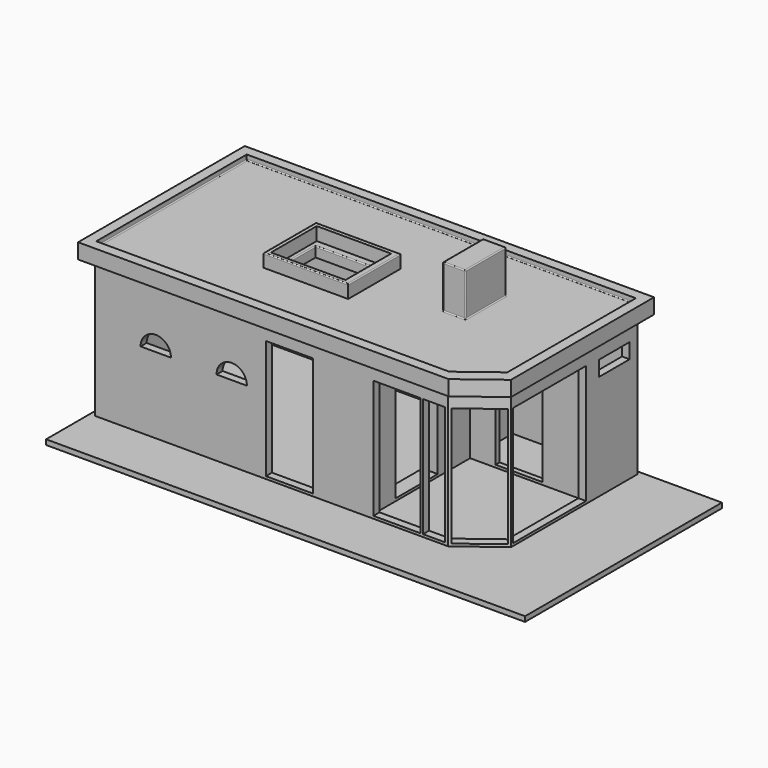
from build123d import *

# Parameters (mm, degrees)
F0_W      = 4950
F0_H      = 3410
F1_DEPTH  = 2700
F2_W      = 930
F2_H      = 2350
F2_W_2    = 434.8470163345
F3_DEPTH  = 159.6687643912
F4_W      = 871.2163103569
F4_H      = 2350
F5_DEPTH  = 182.4564089349
F6_W      = 1800
F6_H      = 2350
F7_DEPTH  = 150
F8_W      = 1040
F8_H      = 2100
F9_DEPTH  = 300
F11_DEPTH = 150
F12_W     = 930
F12_H     = 2100
F13_DEPTH = 100
F14_W     = 700
F14_H     = 240
F15_DEPTH = 1000
F16_W     = 1283.650457859
F16_H     = 300
F17_DEPTH = 300
F18_W     = 9458.89544487
F18_H     = 4860.4282140732
F19_DEPTH = 100
F20_W     = 750
F20_H     = 300
F21_DEPTH = 150
F22_F1_R  = 30
F22_F2_R  = 30
F23_R     = 30
F25_DEPTH = 300
F27_DEPTH = 100
F28_W     = 450
F28_H     = 1000
F29_DEPTH = 850
F32_W     = 1250
F32_H     = 900
F33_DEPTH = 200
F34_W     = 1673.2589006424
F34_H     = 1297.5656241179
F34_W_2   = 1470.5094099045
F34_H_2   = 1129.2519643903
F35_DEPTH = 260
F36_R     = 20
F36_2_R   = 20


# Not quite as in the source:
# - a feature names something its author has since deleted; it is built from what else it names
# - the program builds the solid bodies; features that only make, move or delete a surface that nothing else refers to are left out


with BuildPart() as f1:
    # F0 (on Top) → F1 (new body)
    with BuildSketch(Plane.XY):
        Polygon((-4090.6819343567, 2404.8385477066), (-4090.6819343567, -1305.1614522934), (2885.0078582764, -1305.1614522934), (3659.3180656433, -718.8980095727), (3659.3180656433, 2404.8385477066), align=None)
        with Locations((-1465.6819343567, 549.8385477066)):
            Rectangle(F0_W, F0_H, mode=Mode.SUBTRACT)
        Polygon((1309.3180656433, 1304.8385477066), (1309.3180656433, 2254.8385477066), (3509.3180656433, 2254.8385477066), (3509.3180656433, 1304.8385477066), (3509.3180656433, 1204.8385477066), (3509.3180656433, -625.1614522934), (2809.3180656433, -1155.1614522934), (1309.3180656433, -1155.1614522934), (1309.3180656433, 1204.8385477066), align=None, mode=Mode.SUBTRACT)
        Polygon((1809.3180656433, 1304.8385477066), (1309.3180656433, 1304.8385477066), (1309.3180656433, 1204.8385477066), (1809.3180656433, 1204.8385477066), (3509.3180656433, 1204.8385477066), (3509.3180656433, 1304.8385477066), align=None)
    extrude(amount=F1_DEPTH)

    # F2 (on face) → F3 (cut, through all)
    with BuildSketch(Plane.XZ.offset(1305.1614522934)):
        with BuildLine():
            Line((-1690.6819343567, 1500), (-1090.6819343567, 1500))
            ThreePointArc((-1090.6819343567, 1500), (-1390.6819343567, 1800), (-1690.6819343567, 1500))
        make_face()
        with BuildLine():
            Line((-3190.6819343567, 1500), (-2590.6819343567, 1500))
            ThreePointArc((-2590.6819343567, 1500), (-2890.6819343567, 1800), (-3190.6819343567, 1500))
        make_face()
        with Locations((-251.2006497383, 1225)):
            Rectangle(F2_W, F2_H)
        with Locations((2604.6633028984, 1225)):
            Rectangle(F2_W_2, F2_H)
        with Locations((1872.2397947311, 1225)):
            Rectangle(F2_W, F2_H)
    extrude(amount=-F3_DEPTH, mode=Mode.SUBTRACT)

    # F4 (on face) → F5 (cut, through all)
    with BuildSketch(Plane(origin=(1679.3534909725, -2218.0140446806, 0), x_dir=(0.7972582411, 0.6036383826, 0), z_dir=(0.6036383826, -0.7972582411, 0))):
        with Locations((1997.8588978885, 1225)):
            Rectangle(F4_W, F4_H)
    extrude(amount=-F5_DEPTH, mode=Mode.SUBTRACT)

    # F6 (on face) → F7 (cut, through all)
    with BuildSketch(Plane.YZ.offset(3659.3180656433)):
        with Locations((231.1019904273, 1225)):
            Rectangle(F6_W, F6_H)
    extrude(amount=-F7_DEPTH, mode=Mode.SUBTRACT)

    # F8 (on face) → F9 (cut, through all)
    with BuildSketch(Plane.YZ.offset(1309.3180656433)):
        with Locations((-115.1614522934, 1100)):
            Rectangle(F8_W, F8_H)
    extrude(amount=-F9_DEPTH, mode=Mode.SUBTRACT)

    # F10 (on face) → F11 (cut, through all)
    with BuildSketch(Plane.YZ.offset(-3940.6819343567)):
        with BuildLine():
            Line((1174.8385477066, 1869.0512180328), (1174.8385477066, 0))
            Line((1174.8385477066, 0), (2004.8385477066, 0))
            Line((2004.8385477066, 0), (2004.8385477066, 1869.0512180328))
            ThreePointArc((2004.8385477066, 1869.0512180328), (1589.8385477066, 2284.0512180328), (1174.8385477066, 1869.0512180328))
        make_face()
    extrude(amount=-F11_DEPTH, mode=Mode.SUBTRACT)

    # F12 (on face) → F13 (cut, through all)
    with BuildSketch(Plane.XZ.offset(-1204.8385477066)):
        with Locations((2274.3180656433, 1100)):
            Rectangle(F12_W, F12_H)
    extrude(amount=-F13_DEPTH, mode=Mode.SUBTRACT)

    # F14 (on face) → F15 (join)
    with BuildSketch(Plane.YZ.offset(1309.3180656433)):
        with Locations((704.1475236416, 2454.7141838074)):
            Rectangle(F14_W, F14_H)
    extrude(amount=F15_DEPTH)

    # F16 (on face) → F17 (join)
    with BuildSketch(Plane(origin=(1009.3180656433, 0, 0), x_dir=(0, -1, 0), z_dir=(-1, 0, 0))):
        with Locations((-1055.016964674, 2406.8371295929)):
            Rectangle(F16_W, F16_H)
    extrude(amount=F17_DEPTH)

    # F18 (on face) → F19 (join)
    with BuildSketch(Plane(origin=(0, 0, 0), x_dir=(1, 0, 0), z_dir=(0, 0, -1))):
        with Locations((537.8292798996, -43.6263680458)):
            Rectangle(F18_W, F18_H)
    extrude(amount=F19_DEPTH)

    # F20 (on face) → F21 (cut, through all)
    with BuildSketch(Plane.YZ.offset(3659.3180656433)):
        with Locations((1830.3670287132, 2227.2648965423)):
            Rectangle(F20_W, F20_H)
    extrude(amount=-F21_DEPTH, mode=Mode.SUBTRACT)

    # F22: fillet of radius 30 on 7 edges, made by hand

    # F22_f1
    f22_f1_edges = [f1.edges().sort_by_distance(p)[0] for p in [
        (1809.3180656433, 354.1475236416, 2574.7141838074),
        (1809.3180656433, 354.1475236416, 2334.7141838074),
        (2309.3180656433, 704.1475236416, 2574.7141838074),
        (2309.3180656433, 704.1475236416, 2334.7141838074),
        (1809.3180656433, 1054.1475236416, 2574.7141838074),
        (2309.3180656433, 1054.1475236416, 2454.7141838074),
    ]]
    fillet(f22_f1_edges, radius=F22_F1_R)

    # F22_f2
    f22_f2_edges = [f1.edges().sort_by_distance(p)[0] for p in [
        (1309.3180656433, 704.1475236416, 2574.7141838074),
        (1309.3180656433, 1045.3607270772, 2565.927387243),
        (1309.3180656433, 362.934320206, 2565.927387243),
    ]]
    fillet(f22_f2_edges, radius=F22_F2_R)

    # F23
    f23_edges = [f1.edges().sort_by_distance(p)[0] for p in [
        (709.318066, 1055.016965, 2556.83713),
        (709.318066, 1055.016965, 2256.83713),
        (709.318066, 1696.842194, 2406.83713),
        (709.318066, 413.191736, 2406.83713),
        (859.318066, 413.191736, 2556.83713),
        (859.318066, 413.191736, 2256.83713),
        (859.318066, 1696.842194, 2556.83713),
        (859.318066, 1696.842194, 2256.83713),
    ]]
    fillet(f23_edges, radius=F23_R)

    # F24 (on face) → F25 (join)
    with BuildSketch(Plane.XY.offset(2700)):
        Polygon((3766.5286064148, 2674.4816303253), (-4317.4781799316, 2674.4816303253), (-4317.4781799316, -1439.2734766006), (3001.1787414551, -1439.2734766006), (3766.5286064148, -857.2887182236), align=None)
    extrude(amount=F25_DEPTH)

    # F26 (on face) → F27 (cut)
    with BuildSketch(Plane.XY.offset(3000)):
        Polygon((3566.5286064148, 2474.4816303253), (-4117.4781799316, 2474.4816303253), (-4117.4781799316, -1239.2734766006), (1505.6841762793, -1239.2734766006), (2852.8926372528, -1239.2734766006), (3566.5286064148, -696.6128241371), align=None)
    extrude(amount=-F27_DEPTH, mode=Mode.SUBTRACT)

    # F28 (on face) → F29 (join)
    with BuildSketch(Plane.XY.offset(2900)):
        with Locations((1611.6700674257, 930.6335590078)):
            Rectangle(F28_W, F28_H)
    extrude(amount=F29_DEPTH)

    # F32 (on face) → F33 (cut, through all)
    with BuildSketch(Plane.XY.offset(2900)):
        with Locations((-873.8545744768, 450)):
            Rectangle(F32_W, F32_H)
    extrude(amount=-F33_DEPTH, mode=Mode.SUBTRACT)

    # F36
    f36_edges = [f1.edges().sort_by_distance(p)[0] for p in [
        (1386.670067, 930.633559, 3750),
        (1611.670067, 430.633559, 3750),
        (1611.670067, 1430.633559, 3750),
        (1836.670067, 930.633559, 3750),
        (1836.670067, 430.633559, 3325),
        (1386.670067, 430.633559, 3325),
        (1836.670067, 1430.633559, 3325),
        (3566.528606, 888.934403, 2900),
        (3209.710622, -967.94315, 2900),
        (-275.474787, 2474.48163, 2900),
        (-632.292771, -1239.273477, 2900),
        (-4117.47818, 617.604077, 2900),
        (-873.854574, 900, 2900),
        (-1498.854574, 450, 2900),
        (-873.854574, 0, 2900),
        (-248.854574, 450, 2900),
        (1611.670067, 1430.633559, 2900),
        (1836.670067, 930.633559, 2900),
        (1386.670067, 930.633559, 2900),
        (1611.670067, 430.633559, 2900),
    ]]
    fillet(f36_edges, radius=F36_R)


with BuildPart() as f35:
    # F34 (on face) → F35 (new body)
    with BuildSketch(Plane.XY.offset(2900)):
        with Locations((-836.6294503212, 480.463065207)):
            Rectangle(F34_W, F34_H)
        with Locations((-852.9023528099, 475.8974276483)):
            Rectangle(F34_W_2, F34_H_2, mode=Mode.SUBTRACT)
    extrude(amount=F35_DEPTH)

    # F36#2
    f36_2_edges = [f35.edges().sort_by_distance(p)[0] for p in [
        (0, 480.463065, 3160),
        (-836.62945, -168.319747, 3160),
        (-836.62945, 1129.245877, 3160),
        (-1673.258901, 480.463065, 3160),
    ]]
    fillet(f36_2_edges, radius=F36_2_R)


solid = Compound([f1.part, f35.part])
